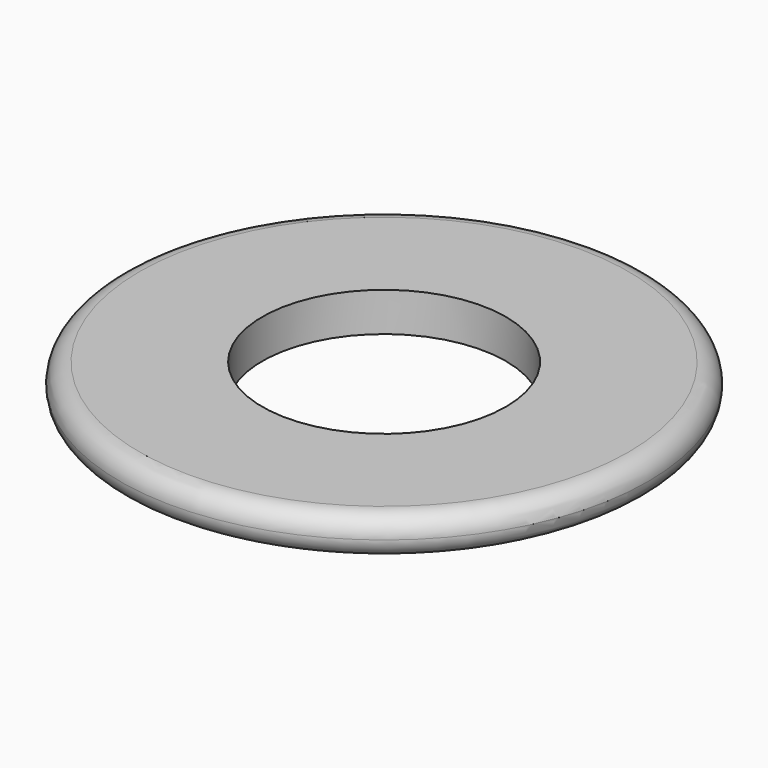
from build123d import *

# Parameters (mm, degrees)
F0_R     = 10.31875
F0_R_2   = 4.7625
F1_DEPTH = 1.524
F2_R     = 0.76199


# Not quite as in the source:
# - a fillet or chamfer is up to 0.001 mm smaller than in the source, because OpenCascade refuses the exact size


with BuildPart() as f1:
    # F0 (on Top) → F1 (new body)
    with BuildSketch(Plane.XY):
        Circle(F0_R)
        Circle(F0_R_2, mode=Mode.SUBTRACT)
    extrude(amount=F1_DEPTH)

    # F2 (radius 0.762 in the source; OpenCascade refuses exactly that, so slightly less here)
    f2_edges = [f1.edges().sort_by_distance(p)[0] for p in [
        (-10.31875, 0, 1.524),
        (-10.31875, 0, 0),
    ]]
    fillet(f2_edges, radius=F2_R)


solid = f1.part
